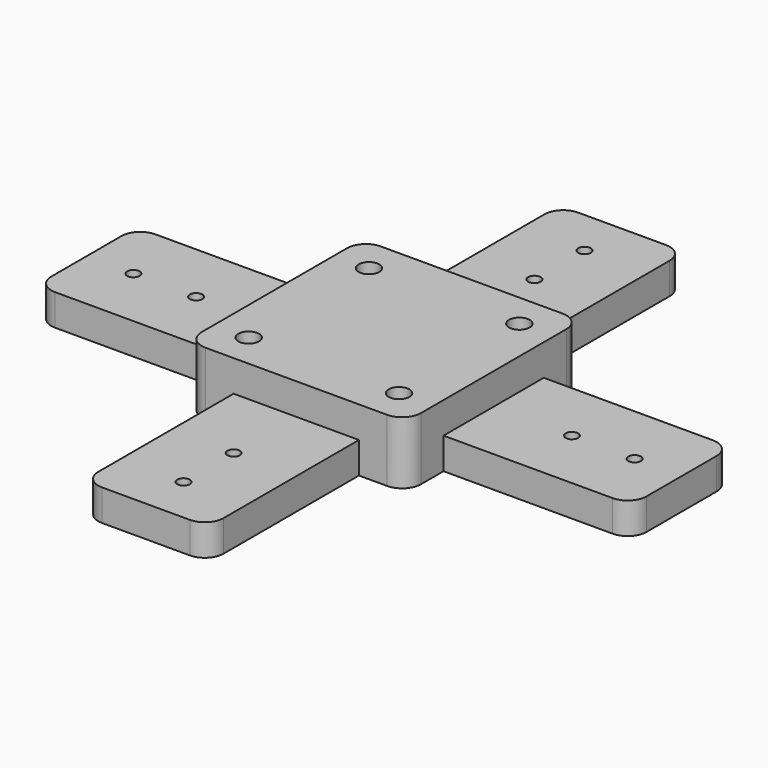
from build123d import *

# Parameters (mm, degrees)
F1_W     = 35
F1_H     = 35
F2_DEPTH = 10
F3_R     = 3
F4_W     = 30
F4_H     = 20
F4_R     = 1
F4_W_2   = 20
F4_H_2   = 30
F5_DEPTH = 5
F6_R     = 3
F8_D     = 3.3


with BuildPart() as f2:
    # F1 (on offset) → F2 (new body)
    with BuildSketch(Plane.XY.offset(9)):
        Rectangle(F1_W, F1_H)
    extrude(amount=F2_DEPTH)

    # F3
    f3_edges = [f2.edges().sort_by_distance(p)[0] for p in [
        (-17.5, -17.5, 14),
        (17.5, -17.5, 14),
        (17.5, 17.5, 14),
        (-17.5, 17.5, 14),
    ]]
    fillet(f3_edges, radius=F3_R)

    # F4 (on offset) → F5 (join)
    with BuildSketch(Plane.XY.offset(9)):
        with Locations((32.5, 0)):
            Rectangle(F4_W, F4_H)
        with Locations((30, 0)):
            Circle(F4_R, mode=Mode.SUBTRACT)
        with Locations((40, 0)):
            Circle(F4_R, mode=Mode.SUBTRACT)
        with Locations((-32.5, 0)):
            Rectangle(F4_W, F4_H)
        with Locations((-40, 0)):
            Circle(F4_R, mode=Mode.SUBTRACT)
        with Locations((-30, 0)):
            Circle(F4_R, mode=Mode.SUBTRACT)
        with Locations((0, -32.5)):
            Rectangle(F4_W_2, F4_H_2)
        with Locations((0, -40)):
            Circle(F4_R, mode=Mode.SUBTRACT)
        with Locations((0, -30)):
            Circle(F4_R, mode=Mode.SUBTRACT)
        with Locations((0, 32.5)):
            Rectangle(F4_W_2, F4_H_2)
        with Locations((0, 30)):
            Circle(F4_R, mode=Mode.SUBTRACT)
        with Locations((0, 40)):
            Circle(F4_R, mode=Mode.SUBTRACT)
    extrude(amount=F5_DEPTH)

    # F6
    f6_edges = [f2.edges().sort_by_distance(p)[0] for p in [
        (-47.5, 10, 11.5),
        (-47.5, -10, 11.5),
        (-10, -47.5, 11.5),
        (10, -47.5, 11.5),
        (47.5, -10, 11.5),
        (47.5, 10, 11.5),
        (10, 47.5, 11.5),
        (-10, 47.5, 11.5),
    ]]
    fillet(f6_edges, radius=F6_R)

    # F8 (through all)
    with Locations(Plane.XY.offset(19)):
        with Locations((-12, 12), (12, 12), (12, -12), (-12, -12)):
            Hole(F8_D / 2)


solid = f2.part
